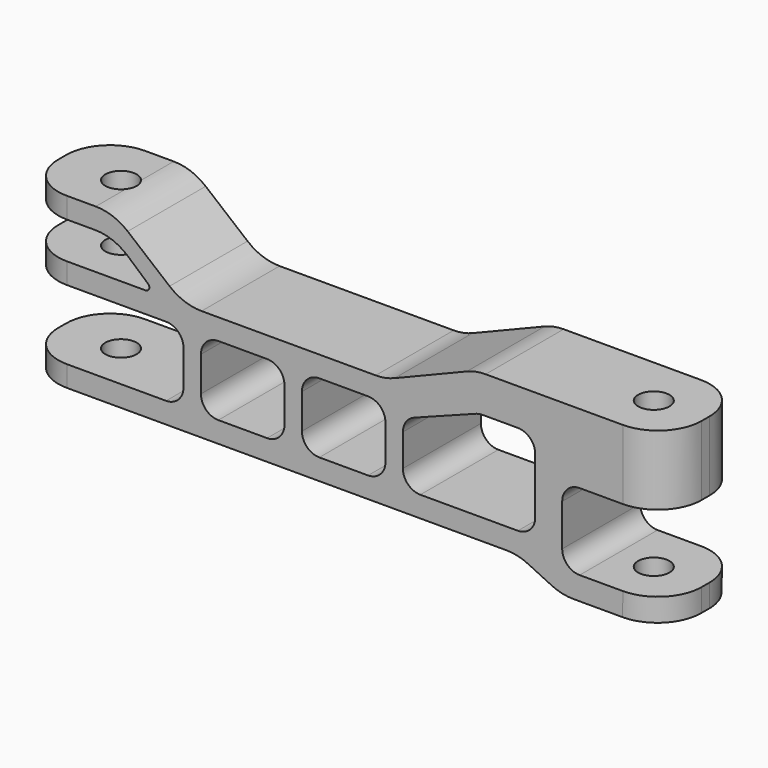
from build123d import *

# Parameters (mm, degrees)
F0_W         = 12
F0_H         = 10
F1_DEPTH     = 14
F2_R         = 2.25
F3_DEPTH     = 99.1
F4_DEPTH     = 25
F5_R         = 6.2769552622
F6_R         = 6.2769552622
F7_R         = 2.5
F8_R         = 2.5
F9_R         = 2.5
F10_R        = 2.5
F11_T1_DEPTH = 14
F11_T3_DEPTH = 21.0473321416
F11_T5_DEPTH = 26.9573104187
F12_R        = 7.2
F13_R        = 7.2
F14_R        = 0.5445837107


# Not quite as in the source:
# - a fillet or chamfer that OpenCascade refuses, or shapes differently, is made with other operations: its cross-section is extruded or revolved along the edge and cut away or added


with BuildPart() as f1:
    # F0 (on Front) → F1 (new body)
    with BuildSketch(Plane.XZ):
        Polygon((59.6290528774, 0), (74.6290528774, 0), (74.6890899837, 3.3114668612), (59.6890899837, 3.3114668612), (59.6890899837, 14.3114668612), (74.6890899837, 14.3114668612), (74.6890899837, 24.3114668612), (47.2866145434, 24.3114668612), (34.3200196198, 19.0325071069), (5.3200196198, 19.0325071069), (-4.6910188856, 27.3114668612), (-17.6799803802, 27.3114668612), (-17.6799803802, 24.3114668612), (-4.6910188856, 24.3114668612), (1.3200196198, 19.0325071069), (-17.6799803802, 19.0325071069), (-17.6799803802, 16.0325071069), (5.3200196198, 16.0325071069), (5.3200196198, 6.0325071069), (-17.6799803802, 6.0325071069), (-17.6799803802, 3.0325071069), (53.3200196198, 3.0325071069), align=None)
        with Locations((13.8200196198, 11.0325071069)):
            Rectangle(F0_W, F0_H, mode=Mode.SUBTRACT)
        with Locations((28.3200196198, 11.0325071069)):
            Rectangle(F0_W, F0_H, mode=Mode.SUBTRACT)
        Polygon((55.8200196198, 6.0325071069), (36.8200196198, 6.0325071069), (36.8200196198, 14.8739311844), (47.7449782193, 19.0325071069), (55.8200196198, 19.0325071069), align=None, mode=Mode.SUBTRACT)
    extrude(amount=F1_DEPTH)

    # F2 (on Top) → F3 (cut)
    with BuildSketch(Plane.XY):
        with Locations((-9.0681398287, -7.2300466709)):
            Circle(F2_R)
        with Locations((67.4190670252, -7.2234715335)):
            Circle(F2_R)
    extrude(amount=F3_DEPTH, mode=Mode.SUBTRACT)

    # F2 (on Top) → F4 (cut)
    with BuildSketch(Plane.XY):
        with Locations((-9.0681398287, -7.2300466709)):
            Circle(F2_R)
        with Locations((67.4190670252, -7.2234715335)):
            Circle(F2_R)
    extrude(amount=-F4_DEPTH, mode=Mode.SUBTRACT)

    # F5
    f5_edges = [f1.edges().sort_by_distance(p)[0] for p in [
        (-17.67998, -14, 25.811467),
        (-17.67998, 0, 25.811467),
        (-17.67998, -14, 17.532507),
        (-17.67998, 0, 17.532507),
        (-17.67998, 0, 4.532507),
        (-17.67998, -14, 4.532507),
    ]]
    fillet(f5_edges, radius=F5_R)

    # F6
    f6_edges = [f1.edges().sort_by_distance(p)[0] for p in [
        (74.68909, -14, 19.311467),
        (74.68909, 0, 19.311467),
        (74.659071, -14, 1.655733),
        (74.659071, 0, 1.655733),
    ]]
    fillet(f6_edges, radius=F6_R)

    # F7
    f7_edges = [f1.edges().sort_by_distance(p)[0] for p in [
        (36.82002, -7, 6.032507),
        (36.82002, -7, 14.873931),
        (47.744978, -7, 19.032507),
        (55.82002, -7, 19.032507),
        (55.82002, -7, 6.032507),
    ]]
    fillet(f7_edges, radius=F7_R)

    # F8
    f8_edges = [f1.edges().sort_by_distance(p)[0] for p in [
        (34.32002, -7, 16.032507),
        (22.32002, -7, 16.032507),
        (22.32002, -7, 6.032507),
        (34.32002, -7, 6.032507),
    ]]
    fillet(f8_edges, radius=F8_R)

    # F9
    f9_edges = [f1.edges().sort_by_distance(p)[0] for p in [
        (19.82002, -7, 16.032507),
        (7.82002, -7, 16.032507),
        (7.82002, -7, 6.032507),
        (19.82002, -7, 6.032507),
    ]]
    fillet(f9_edges, radius=F9_R)

    # F10
    f10_edges = [f1.edges().sort_by_distance(p)[0] for p in [
        (5.32002, -7, 16.032507),
        (5.32002, -7, 6.032507),
        (59.68909, -7, 14.311467),
        (59.68909, -7, 3.311467),
    ]]
    fillet(f10_edges, radius=F10_R)

    # F11: fillet of radius 7.2 on 4 edges, made by hand

    # F11_s2 → F11_t1 (join)
    with BuildSketch(Plane.XZ):
        with BuildLine():
            ThreePointArc((35.6254467793, 19.5639725748), (34.2937652809, 19.1666225681), (32.9105531914, 19.0325071069))
            Line((32.9105531914, 19.0325071069), (34.3200196198, 19.0325071069))
            Line((34.3200196198, 19.0325071069), (35.6254467793, 19.5639725748))
        make_face()
        with BuildLine():
            ThreePointArc((7.9114817035, 19.0325071069), (5.4731495991, 19.457956454), (3.3229804953, 20.6840247322))
            Line((3.3229804953, 20.6840247322), (5.3200196198, 19.0325071069))
            Line((5.3200196198, 19.0325071069), (7.9114817035, 19.0325071069))
        make_face()
    extrude(amount=F11_T1_DEPTH)

    # F11_s4 → F11_t3 (cut)
    with BuildSketch(Plane.XZ.offset(-3.5236660708)):
        with BuildLine():
            ThreePointArc((48.6960809717, 24.3114668612), (47.3128688823, 24.1773514), (45.9811873838, 23.7800013933))
            Line((45.9811873838, 23.7800013933), (47.2866145434, 24.3114668612))
            Line((47.2866145434, 24.3114668612), (48.6960809717, 24.3114668612))
        make_face()
    extrude(amount=F11_T3_DEPTH, mode=Mode.SUBTRACT)

    # F11_s6 → F11_t5 (cut)
    with BuildSketch(Plane.XZ.offset(-6.4786552093)):
        with BuildLine():
            ThreePointArc((-2.6939797611, 25.6599492359), (-4.844148865, 26.8860175141), (-7.2824809693, 27.3114668612))
            Line((-7.2824809693, 27.3114668612), (-4.6910188856, 27.3114668612))
            Line((-4.6910188856, 27.3114668612), (-2.6939797611, 25.6599492359))
        make_face()
    extrude(amount=F11_T5_DEPTH, mode=Mode.SUBTRACT)

    # F12
    f12_edges = [f1.edges().sort_by_distance(p)[0] for p in [
        (53.32002, -7, 3.032507),
        (59.629053, -7, 0),
    ]]
    fillet(f12_edges, radius=F12_R)

    # F13
    f13_edges = [f1.edges().sort_by_distance(p)[0] for p in [
        (-4.691019, -7, 24.311467),
    ]]
    fillet(f13_edges, radius=F13_R)

    # F14
    f14_edges = [f1.edges().sort_by_distance(p)[0] for p in [
        (1.32002, -7, 19.032507),
    ]]
    fillet(f14_edges, radius=F14_R)


solid = f1.part
